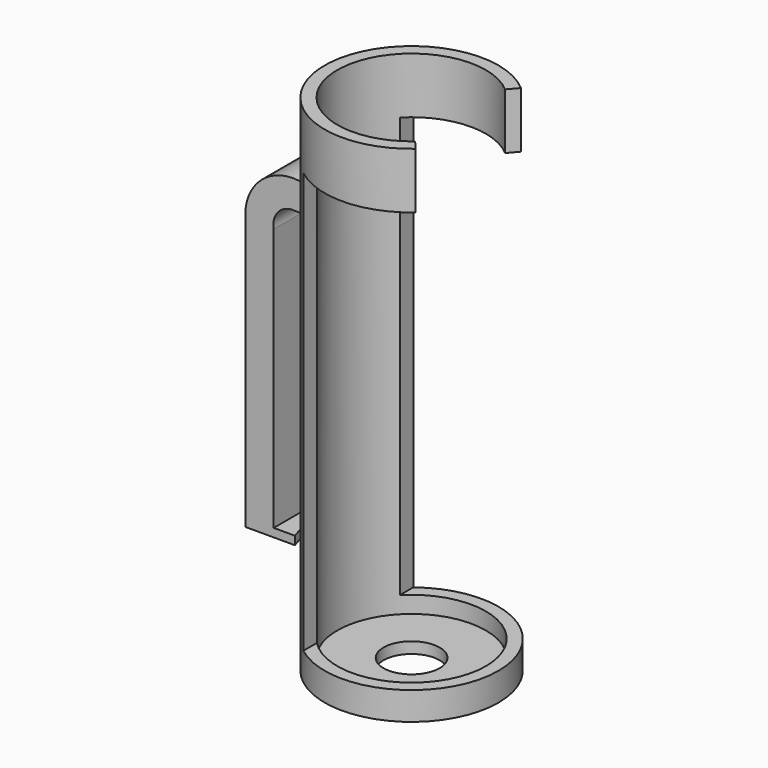
from build123d import *

# Parameters (mm, degrees)
F0_R      = 15.5
F0_R_2    = 13.25
F1_DEPTH  = 90
F2_R      = 15.5
F3_DEPTH  = 2
F4_R      = 5
F5_DEPTH  = 90.001
F6_W      = 25
F6_H      = 75
F7_DEPTH  = 30
F9_DEPTH  = 6
F10_W     = 5.0829965621
F10_H     = 1.5
F11_DEPTH = 6
F13_DEPTH = 25
F15_DEPTH = 25
F16_DEPTH = 25


# Not quite as in the source:
# - a feature names something its author has since deleted; it is built from what else it names


with BuildPart() as f1:
    # F0 (on Top) → F1 (new body)
    with BuildSketch(Plane.XY):
        Circle(F0_R)
        Circle(F0_R_2, mode=Mode.SUBTRACT)
    extrude(amount=F1_DEPTH)

    # F2 (on Top) → F3 (join)
    with BuildSketch(Plane.XY):
        Circle(F2_R)
    extrude(amount=F3_DEPTH)

    # F4 (on Top) → F5 (cut, through all)
    with BuildSketch(Plane.XY):
        Circle(F4_R)
    extrude(amount=F5_DEPTH, mode=Mode.SUBTRACT)

    # F6 (on Front) → F7 (cut, symmetric)
    with BuildSketch(Plane.XZ):
        with Locations((3, 42.5)):
            Rectangle(F6_W, F6_H)
    extrude(amount=F7_DEPTH, both=True, mode=Mode.SUBTRACT)

    # F8 (on Front) → F9 (join, symmetric)
    with BuildSketch(Plane.XZ):
        with BuildLine():
            Line((-14.3252154812, 74.3832364678), (-15.3322340921, 74.3832364678))
            ThreePointArc((-15.3322340921, 74.3832364678), (-22.3824376382, 71.9712620232), (-24.7944127768, 64.9210587144))
            Line((-24.7944127768, 64.9210587144), (-24.7944127768, 16.9092640281))
            Line((-24.7944127768, 16.9092640281), (-19.7944119573, 16.9092640281))
            Line((-19.7944119573, 16.9092640281), (-19.7944119573, 65.3066100025))
            ThreePointArc((-19.7944119573, 65.3066100025), (-18.9325593375, 68.3469659349), (-15.9612301203, 69.4229570209))
            Line((-15.9612301203, 69.4229570209), (-14.3252154812, 69.4229570209))
            Line((-14.3252154812, 69.4229570209), (-14.3252154812, 74.3832364678))
        make_face()
    extrude(amount=F9_DEPTH, both=True)

    # F10 (on Front) → F11 (join, symmetric)
    with BuildSketch(Plane.XZ):
        with BuildLine():
            Line((-14.3252154812, 74.3832364678), (-15.3322340921, 74.3832364678))
            ThreePointArc((-15.3322340921, 74.3832364678), (-22.3824376382, 71.9712620232), (-24.7944127768, 64.9210587144))
            Line((-24.7944127768, 64.9210587144), (-24.7944127768, 16.9092640281))
            Line((-24.7944127768, 16.9092640281), (-19.7944119573, 16.9092640281))
            Line((-19.7944119573, 16.9092640281), (-19.7944119573, 18.4092640281))
            Line((-19.7944119573, 18.4092640281), (-19.7944119573, 65.3066100025))
            ThreePointArc((-19.7944119573, 65.3066100025), (-18.9325593375, 68.3469659349), (-15.9612301203, 69.4229570209))
            Line((-15.9612301203, 69.4229570209), (-14.3252154812, 69.4229570209))
            Line((-14.3252154812, 69.4229570209), (-14.3252154812, 74.3832364678))
        make_face()
        with Locations((-17.2529136762, 17.6592640281)):
            Rectangle(F10_W, F10_H)
    extrude(amount=F11_DEPTH, both=True)

    # F12 (on Top) → F13 (cut)
    with BuildSketch(Plane.XY):
        with BuildLine():
            Line((-13.8731463173, 7.0058838464), (-15.6120072238, 7.0058838464))
            ThreePointArc((-15.6120072238, 7.0058838464), (-17.1111072391, 0.1648850375), (-15.74411501, -6.7037318396))
            Line((-15.74411501, -6.7037318396), (-14.0216467162, -6.7037318396))
            ThreePointArc((-14.0216467162, -6.7037318396), (-15.5408577678, 0.1683361248), (-13.8731463173, 7.0058838464))
        make_face()
    extrude(amount=F13_DEPTH, mode=Mode.SUBTRACT)

    # F14 (on face) → F15 (cut)
    with BuildSketch(Plane.XY.offset(90)):
        with BuildLine():
            Line((11.193397513, 12.9792110231), (0, 0))
            Line((0, 0), (11.193397513, -12.9792110231))
            ThreePointArc((11.193397513, -12.9792110231), (17.1391967918, 0), (11.193397513, 12.9792110231))
        make_face()
    extrude(amount=-F15_DEPTH, mode=Mode.SUBTRACT)

    # F14 (on face) → F16 (cut)
    with BuildSketch(Plane.XY.offset(90)):
        with BuildLine():
            Line((10.1228583556, 11.7378762437), (8.6534111749, 10.0339909826))
            ThreePointArc((8.6534111749, 10.0339909826), (12.0461653249, 5.5183694119), (13.25, 0))
            ThreePointArc((13.25, 0), (12.0461653249, -5.5183694119), (8.6534111749, -10.0339909826))
            Line((8.6534111749, -10.0339909826), (10.1228583556, -11.7378762437))
            ThreePointArc((10.1228583556, -11.7378762437), (14.0917405687, -6.4554510102), (15.5, 0))
            ThreePointArc((15.5, 0), (14.0917405687, 6.4554510102), (10.1228583556, 11.7378762437))
        make_face()
        with BuildLine():
            Line((11.193397513, 12.9792110231), (10.1228583556, 11.7378762437))
            ThreePointArc((10.1228583556, 11.7378762437), (14.0917405687, 6.4554510102), (15.5, 0))
            ThreePointArc((15.5, 0), (14.0917405687, -6.4554510102), (10.1228583556, -11.7378762437))
            Line((10.1228583556, -11.7378762437), (11.193397513, -12.9792110231))
            ThreePointArc((11.193397513, -12.9792110231), (17.1391967918, 0), (11.193397513, 12.9792110231))
        make_face()
        with BuildLine():
            Line((8.6534111749, 10.0339909826), (0, 0))
            Line((0, 0), (8.6534111749, -10.0339909826))
            ThreePointArc((8.6534111749, -10.0339909826), (12.0461653249, -5.5183694119), (13.25, 0))
            ThreePointArc((13.25, 0), (12.0461653249, 5.5183694119), (8.6534111749, 10.0339909826))
        make_face()
    extrude(amount=-F16_DEPTH, mode=Mode.SUBTRACT)


solid = f1.part
